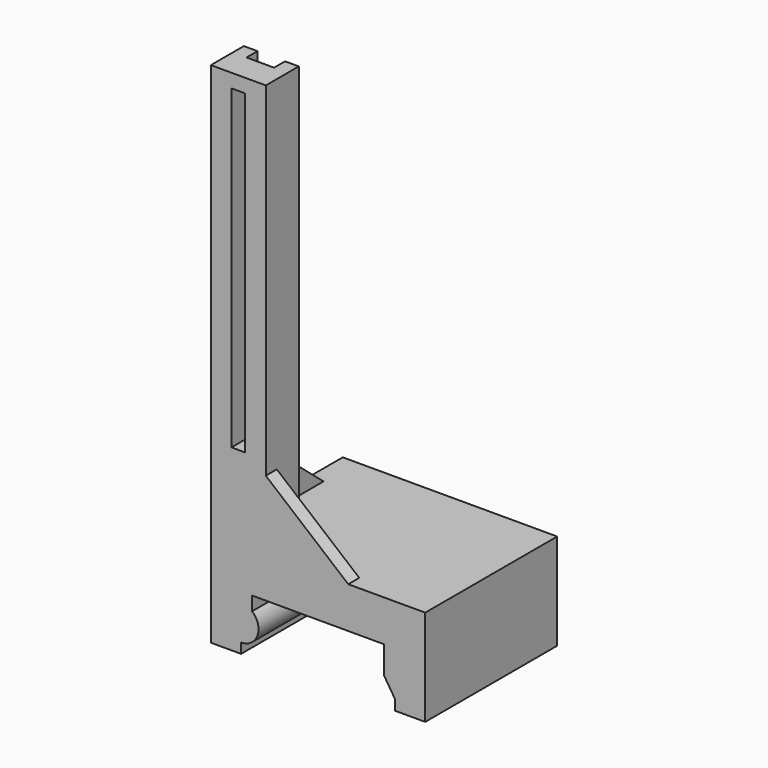
from build123d import *

# Parameters (mm, degrees)
F1_DEPTH  = 38.1
F2_W      = 71.12
F2_H      = 27.3908400369
F3_DEPTH  = 50.8
F4_W      = 25.4
F4_H      = 19.05
F5_DEPTH  = 190.5
F6_W      = 12.7
F6_H      = 152.4
F7_DEPTH  = 6.35
F9_DEPTH  = 6.35
F10_R     = 8.0648205789
F11_DEPTH = 76.2
F13_DEPTH = 76.2
F15_DEPTH = 6.35
F17_DEPTH = 6.35
F18_W     = 6.35
F18_H     = 146.05
F19_DEPTH = 25.4


with BuildPart() as f1:
    # F0 (on Front) → F1 (new body, symmetric)
    with BuildSketch(Plane.XZ):
        Polygon((30.48, -22.225), (49.53, -22.225), (49.53, 22.225), (-49.53, 22.225), (-49.53, -22.225), (-30.48, -22.225), (-30.48, 3.175), (30.48, 3.175), align=None)
    extrude(amount=F1_DEPTH, both=True)

    # F2 (on Front) → F3 (cut, symmetric)
    with BuildSketch(Plane.XZ):
        with Locations((0, -23.2204200185)):
            Rectangle(F2_W, F2_H)
    extrude(amount=F3_DEPTH, both=True, mode=Mode.SUBTRACT)

    # F4 (on face) → F5 (join)
    with BuildSketch(Plane.XY.offset(22.225)):
        with Locations((-36.83, -28.575)):
            Rectangle(F4_W, F4_H)
    extrude(amount=F5_DEPTH)

    # F6 (on face) → F7 (cut)
    with BuildSketch(Plane(origin=(0, -19.05, 0), x_dir=(-1, 0, 0), z_dir=(0, 1, 0))):
        with Locations((36.83, 136.525)):
            Rectangle(F6_W, F6_H)
    extrude(amount=-F7_DEPTH, mode=Mode.SUBTRACT)

    # F8 (on face) → F9 (cut)
    with BuildSketch(Plane(origin=(0, -19.05, 0), x_dir=(-1, 0, 0), z_dir=(0, 1, 0))):
        Polygon((33.655, 200.025), (33.655, 225.425), (20.955, 225.425), (20.955, 200.025), (24.13, 200.025), (24.13, 212.725), (30.48, 212.725), (30.48, 200.025), align=None)
    extrude(amount=-F9_DEPTH, mode=Mode.SUBTRACT)

    # F10 (on face) → F11 (join)
    with BuildSketch(Plane.XZ.offset(38.1)):
        with Locations((-35.56, -9.525)):
            Circle(F10_R)
    extrude(amount=-F11_DEPTH)

    # F12 (on face) → F13 (join)
    with BuildSketch(Plane.XZ.offset(38.1)):
        Polygon((35.56, -17.4720194191), (35.56, -9.525), (30.48, -9.525), align=None)
    extrude(amount=-F13_DEPTH)

    # F14 (on face) → F15 (join)
    with BuildSketch(Plane.XZ.offset(38.1)):
        Polygon((-24.13, 53.975), (-24.13, 22.225), (13.97, 22.225), align=None)
    extrude(amount=-F15_DEPTH)

    # F16 (on face) → F17 (join)
    with BuildSketch(Plane(origin=(-49.53, 0, 0), x_dir=(0, -1, 0), z_dir=(-1, 0, 0))):
        Polygon((-19.05, 22.225), (19.05, 22.225), (19.05, 53.975), align=None)
    extrude(amount=-F17_DEPTH)

    # F18 (on face) → F19 (cut)
    with BuildSketch(Plane.XZ.offset(38.1)):
        with Locations((-36.83, 133.35)):
            Rectangle(F18_W, F18_H)
    extrude(amount=-F19_DEPTH, mode=Mode.SUBTRACT)


solid = f1.part
